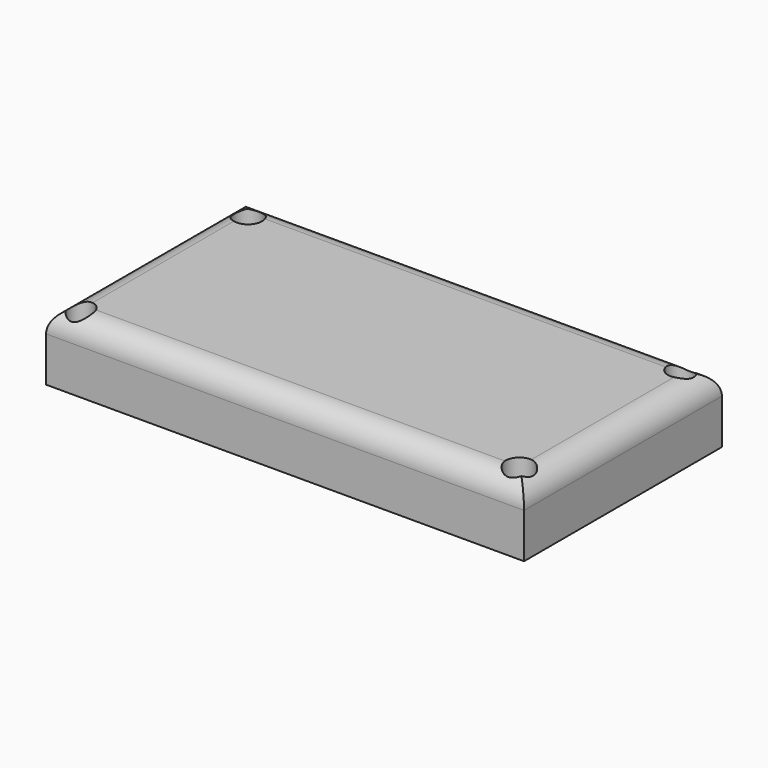
from build123d import *

# Parameters (mm, degrees)
F0_W        = 106.775932014
F0_H        = 55.2587080747
F0_R        = 2.7303671047
F0_R_2      = 3.1130972935
F0_R_3      = 3.09976381
F0_R_4      = 2.8780568391
F1_DEPTH    = 15
F2_T1_DEPTH = 131.775932014
F2_T3_DEPTH = 80.2587080747


# Not quite as in the source:
# - a fillet or chamfer that OpenCascade refuses, or shapes differently, is made with other operations: its cross-section is extruded or revolved along the edge and cut away or added


with BuildPart() as f1:
    # F0 (on Top) → F1 (new body)
    with BuildSketch(Plane.XY):
        with Locations((6.0439184308, 7.6268529519)):
            Rectangle(F0_W, F0_H)
        with Locations((-42.7391566336, -15.973219648)):
            Circle(F0_R, mode=Mode.SUBTRACT)
        with Locations((54.2513802648, -14.8219969124)):
            Circle(F0_R_2, mode=Mode.SUBTRACT)
        with Locations((-41.587933898, 29.2122848332)):
            Circle(F0_R_3, mode=Mode.SUBTRACT)
        with Locations((53.6757707596, 30.9391189367)):
            Circle(F0_R_4, mode=Mode.SUBTRACT)
    extrude(amount=F1_DEPTH)

    # F2: fillet of radius 5 on 4 edges, made by hand

    # F2_s2 → F2_t1 (cut)
    with BuildSketch(Plane.YZ.offset(-59.8440475762)):
        with BuildLine():
            ThreePointArc((-20.0025010854, 10), (-18.5380349913, 13.5355339059), (-15.0025010854, 15))
            Line((-15.0025010854, 15), (-20.0025010854, 15))
            Line((-20.0025010854, 15), (-20.0025010854, 10))
        make_face()
        with BuildLine():
            ThreePointArc((35.2562069893, 10), (33.7917408952, 13.5355339059), (30.2562069893, 15))
            Line((30.2562069893, 15), (35.2562069893, 15))
            Line((35.2562069893, 15), (35.2562069893, 10))
        make_face()
    extrude(amount=F2_T1_DEPTH, mode=Mode.SUBTRACT)

    # F2_s4 → F2_t3 (cut)
    with BuildSketch(Plane.XZ.offset(-47.7562069893)):
        with BuildLine():
            ThreePointArc((59.4318844378, 10), (57.9674183437, 13.5355339059), (54.4318844378, 15))
            Line((54.4318844378, 15), (59.4318844378, 15))
            Line((59.4318844378, 15), (59.4318844378, 10))
        make_face()
        with BuildLine():
            ThreePointArc((-47.3440475762, 10), (-45.8795814821, 13.5355339059), (-42.3440475762, 15))
            Line((-42.3440475762, 15), (-47.3440475762, 15))
            Line((-47.3440475762, 15), (-47.3440475762, 10))
        make_face()
    extrude(amount=F2_T3_DEPTH, mode=Mode.SUBTRACT)


solid = f1.part
